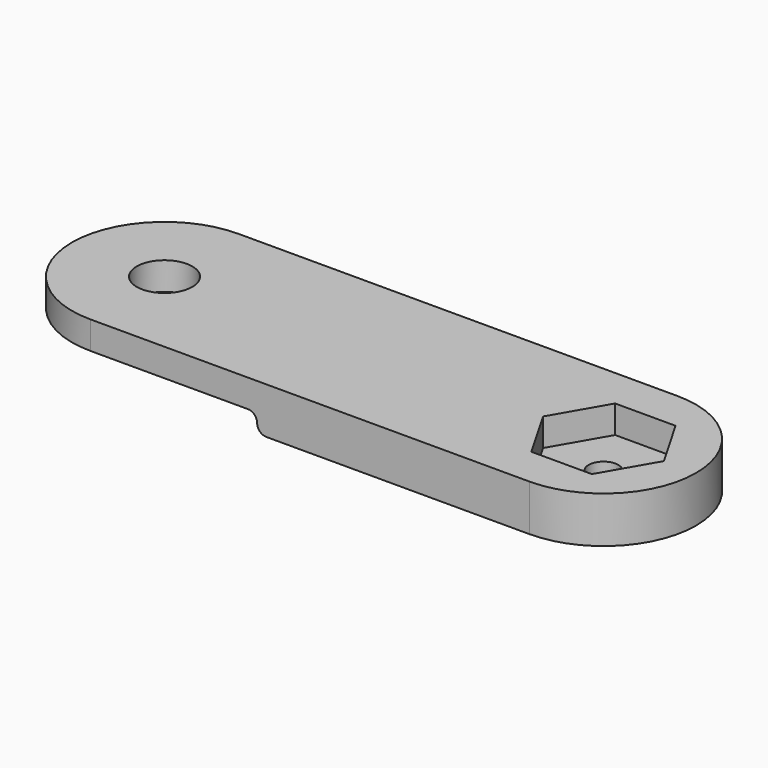
from build123d import *

# Parameters (mm, degrees)
F0_R     = 3
F1_DEPTH = 5
F0_R_2   = 1.6
F2_DEPTH = 2
F4_W     = 30
F4_H     = 20
F5_DEPTH = 2
F6_R     = 0.99999


# Not quite as in the source:
# - a fillet or chamfer is up to 0.001 mm smaller than in the source, because OpenCascade refuses the exact size


with BuildPart() as f1:
    # F0 (on Top) → F1 (new body)
    with BuildSketch(Plane.XY):
        with BuildLine():
            Line((-47.4, -10), (0, -10))
            ThreePointArc((0, -10), (10, 0), (0, 10))
            Line((0, 10), (-47.4, 10))
            ThreePointArc((-47.4, 10), (-57.4, 0), (-47.4, -10))
        make_face()
        with Locations((-47.4, 0)):
            Circle(F0_R, mode=Mode.SUBTRACT)
        Polygon((-6.5240580418, 0), (-3.2620290209, 5.65), (3.2620290209, 5.65), (6.5240580418, 0), (3.2620290209, -5.65), (-3.2620290209, -5.65), align=None, mode=Mode.SUBTRACT)
    extrude(amount=F1_DEPTH)

    # F0 (on Top) → F2 (join)
    with BuildSketch(Plane.XY):
        Polygon((3.2620290209, 5.65), (-3.2620290209, 5.65), (-6.5240580418, 0), (-3.2620290209, -5.65), (3.2620290209, -5.65), (6.5240580418, 0), align=None)
        Circle(F0_R_2, mode=Mode.SUBTRACT)
    extrude(amount=F2_DEPTH)

    # F4 (on face) → F5 (cut)
    with BuildSketch(Plane(origin=(0, 0, 0), x_dir=(1, 0, 0), z_dir=(0, 0, -1))):
        with Locations((-44.4, 0)):
            Rectangle(F4_W, F4_H)
    extrude(amount=-F5_DEPTH, mode=Mode.SUBTRACT)

    # F6 (radius 1 in the source; OpenCascade refuses exactly that, so slightly less here)
    f6_edges = [f1.edges().sort_by_distance(p)[0] for p in [
        (-29.4, 0, 2),
        (-29.4, 0, 0),
    ]]
    fillet(f6_edges, radius=F6_R)


solid = f1.part
